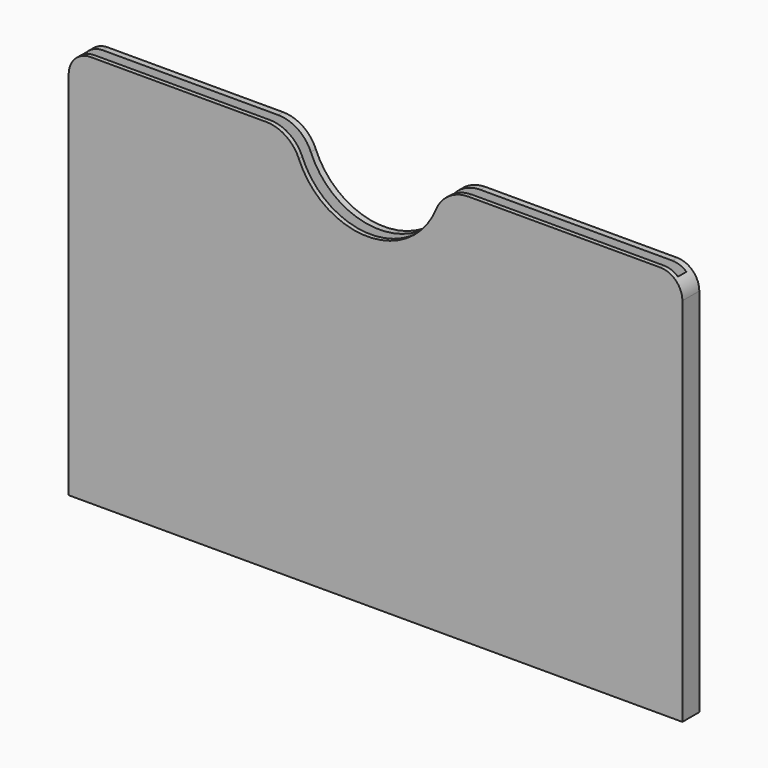
from build123d import *

# Parameters (mm, degrees)
F0_W        = 87
F0_H        = 3
F0_W_2      = 85
F0_H_2      = 1.5
F1_DEPTH    = 54.5
F3_DEPTH    = 10
F4_T1_DEPTH = 18.6923881554
F5_T1_DEPTH = 18.69
F6_W        = 87
F6_H        = 3
F7_DEPTH    = 1.2
F8_R        = 5


# Not quite as in the source:
# - a fillet or chamfer that OpenCascade refuses, or shapes differently, is made with other operations: its cross-section is extruded or revolved along the edge and cut away or added


with BuildPart() as f1:
    # F0 (on Top) → F1 (new body)
    with BuildSketch(Plane.XY):
        with Locations((18.8151740879, 14.6483827978)):
            Rectangle(F0_W, F0_H)
        with Locations((18.7021535635, 14.5136903673)):
            Rectangle(F0_W_2, F0_H_2, mode=Mode.SUBTRACT)
    extrude(amount=F1_DEPTH)

    # F2 (on face) → F3 (cut)
    with BuildSketch(Plane.XZ.offset(-13.1483827978)):
        with BuildLine():
            Line((28.1252544373, 54.5), (7.2028026916, 54.5))
            ThreePointArc((7.2028026916, 54.5), (17.6640285645, 44.8635037778), (28.1252544373, 54.5))
        make_face()
    extrude(amount=-F3_DEPTH, mode=Mode.SUBTRACT)

    # F4: fillet of radius 3.1384776311 on 1 edges, made by hand

    # F4_s2 → F4_t1 (cut)
    with BuildSketch(Plane.XZ.offset(-23.9945768755)):
        with BuildLine():
            ThreePointArc((59.1766964568, 54.5), (61.3959352723, 53.5807611845), (62.3151740879, 51.3615223689))
            Line((62.3151740879, 51.3615223689), (62.3151740879, 54.5))
            Line((62.3151740879, 54.5), (59.1766964568, 54.5))
        make_face()
    extrude(amount=F4_T1_DEPTH, mode=Mode.SUBTRACT)

    # F5: fillet of radius 3.138 on 1 edges, made by hand

    # F5_s2 → F5_t1 (cut)
    with BuildSketch(Plane.XZ.offset(-23.9933827978)):
        with BuildLine():
            ThreePointArc((-24.6848259121, 51.362), (-23.7657269915, 53.5809010794), (-21.5468259121, 54.5))
            Line((-21.5468259121, 54.5), (-24.6848259121, 54.5))
            Line((-24.6848259121, 54.5), (-24.6848259121, 51.362))
        make_face()
    extrude(amount=F5_T1_DEPTH, mode=Mode.SUBTRACT)

    # F6 (on Top) → F7 (join)
    with BuildSketch(Plane.XY):
        with Locations((18.8151740879, 14.6483827978)):
            Rectangle(F6_W, F6_H)
    extrude(amount=-F7_DEPTH)

    # F8
    f8_edges = [f1.edges().sort_by_distance(p)[0] for p in [
        (28.125254, 13.456037, 54.5),
        (28.125254, 15.706037, 54.5),
        (7.202803, 13.456037, 54.5),
        (7.202803, 15.706037, 54.5),
    ]]
    fillet(f8_edges, radius=F8_R)


solid = f1.part
